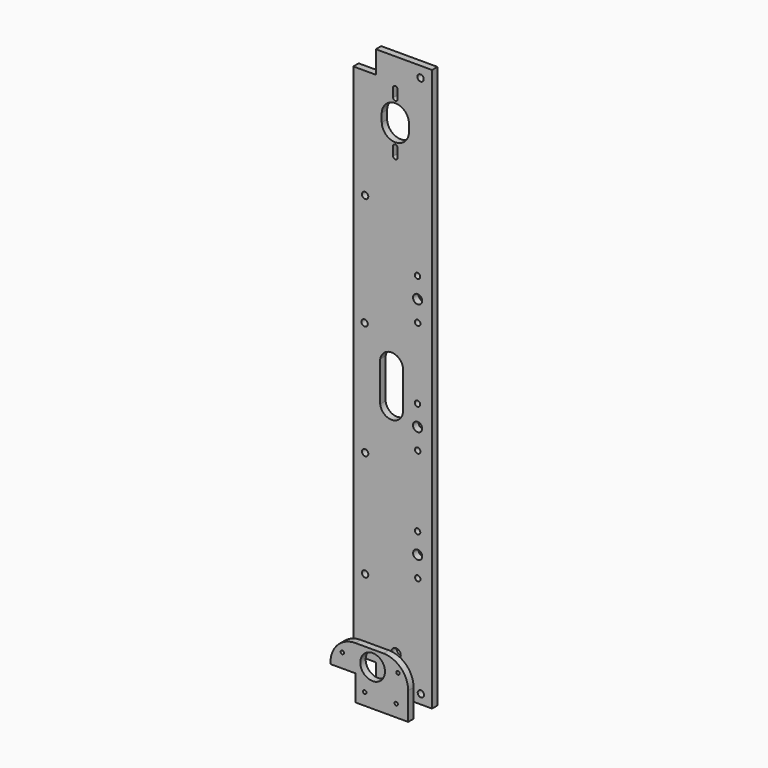
from build123d import *

# Parameters (mm, degrees)
F0_R     = 2.8321056642
F0_R_2   = 2.8346456693
F0_R_3   = 4.2506985014
F0_R_4   = 2.4282448565
F0_R_5   = 4.0601981204
F0_R_6   = 2.4234188468
F0_R_7   = 2.8384556769
F0_R_8   = 2.8333756668
F1_DEPTH = 6
F3_R     = 1.5196800403
F3_R_2   = 1.5209496142
F3_R_3   = 11
F4_DEPTH = 6


# Not quite as in the source:
# - ends of sketch curves that miss each other by under 0.0002 mm in the source are joined


with BuildPart() as f1:
    # F0 (on Front) → F1 (new body)
    with BuildSketch(Plane.XZ):
        Polygon((-15.0012700025, 250), (-15.0012700025, 230), (-34.9987299975, 230), (-34.9987299975, -230), (-15.0012700025, -230), (-15.0012700025, -250), (34.9987299975, -250), (34.9987299975, 250), align=None)
        with Locations((-24.5161290323, -163.967487935)):
            Circle(F0_R, mode=Mode.SUBTRACT)
        with Locations((-24.5161290323, -68.9585979172)):
            Circle(F0_R_2, mode=Mode.SUBTRACT)
        with BuildLine():
            ThreePointArc((-11.0922101342, 8.6664987085), (-0.9906019812, 17.1704343409), (9.1110061718, 8.6664987085))
            Line((9.1110061718, 8.6664987085), (9.110998222, -26.6289052578))
            ThreePointArc((9.110998222, -26.6289052578), (-0.9906019812, -35.5824231648), (-11.0922037581, -26.6289054481))
            Line((-11.0922037581, -26.6289054481), (-11.0922101342, 8.6664987085))
        make_face(mode=Mode.SUBTRACT)
        with Locations((2.9337058674, -217.3037846076)):
            Circle(F0_R_3, mode=Mode.SUBTRACT)
        with Locations((25.0952501905, -241.6408432817)):
            Circle(F0_R_2, mode=Mode.SUBTRACT)
        with Locations((22.3344424689, -152.1221742443)):
            Circle(F0_R_4, mode=Mode.SUBTRACT)
        with Locations((22.2428244856, -133.6652273305)):
            Circle(F0_R_5, mode=Mode.SUBTRACT)
        with Locations((22.1522987046, -115.4320548641)):
            Circle(F0_R_6, mode=Mode.SUBTRACT)
        with Locations((22.2455422911, -52.1094742189)):
            Circle(F0_R_4, mode=Mode.SUBTRACT)
        with Locations((22.1539243078, -33.6525273051)):
            Circle(F0_R_5, mode=Mode.SUBTRACT)
        with Locations((22.0633985268, -15.4193548387)):
            Circle(F0_R_6, mode=Mode.SUBTRACT)
        with Locations((-24.953009906, 32.4752349505)):
            Circle(F0_R_7, mode=Mode.SUBTRACT)
        with Locations((-24.5161290323, 132.3888747777)):
            Circle(F0_R_8, mode=Mode.SUBTRACT)
        with Locations((22.2455422911, 47.904495809)):
            Circle(F0_R_4, mode=Mode.SUBTRACT)
        with Locations((22.1539243078, 66.3614427229)):
            Circle(F0_R_5, mode=Mode.SUBTRACT)
        with Locations((22.0633985268, 84.5946151892)):
            Circle(F0_R_6, mode=Mode.SUBTRACT)
        with BuildLine():
            ThreePointArc((0.322589783, 179.2583173603), (2.3685547371, 181.0616967234), (4.4145196912, 179.2583173603))
            Line((4.4145196912, 179.2583173603), (4.4145288291, 171.2014224028))
            ThreePointArc((4.4145288291, 171.2014224028), (2.3685547371, 169.395478791), (0.3225807849, 171.2014224203))
            Line((0.3225807849, 171.2014224203), (0.322589783, 179.2583173603))
        make_face(mode=Mode.SUBTRACT)
        with BuildLine():
            ThreePointArc((-9.7358355642, 201.8008634341), (2.3672847346, 213.3959613919), (14.4704050333, 201.8008634341))
            Line((14.4704050333, 201.8008634341), (14.4704089408, 194.3281686563))
            ThreePointArc((14.4704089408, 194.3281686563), (2.3672847346, 182.730480061), (-9.735849035, 194.3281682483))
            Line((-9.735849035, 194.3281682483), (-9.7358355642, 201.8008634341))
        make_face(mode=Mode.SUBTRACT)
        with BuildLine():
            ThreePointArc((0.322589783, 225.0952490342), (2.3685547371, 226.8986283973), (4.4145196912, 225.0952490342))
            Line((4.4145196912, 225.0952490342), (4.4145288291, 217.0383540767))
            ThreePointArc((4.4145288291, 217.0383540767), (2.3685547371, 215.2324104648), (0.3225807849, 217.0383540942))
            Line((0.3225807849, 217.0383540942), (0.322589783, 225.0952490342))
        make_face(mode=Mode.SUBTRACT)
        with Locations((24.7548895098, 240.3987807976)):
            Circle(F0_R_2, mode=Mode.SUBTRACT)
    extrude(amount=F1_DEPTH)


with BuildPart() as f4:
    # F3 (on offset) → F4 (new body)
    with BuildSketch(Plane.XZ.offset(26)):
        with BuildLine():
            Line((-34.429923848, -225.4829136519), (-34.429923848, -227.1858596432))
            Line((-34.429923848, -227.1858596432), (-12.0509845344, -227.1858596432))
            Line((-12.0509845344, -227.1858596432), (-12.0509845344, -249.9848689689))
            Line((-12.0509845344, -249.9848689689), (34.579038782, -249.9848689689))
            Line((34.579038782, -249.9848689689), (34.579038782, -225.4829136519))
            ThreePointArc((34.579038782, -225.4829136519), (28.1353879681, -209.9265644658), (12.579038782, -203.4829136519))
            Line((12.579038782, -203.4829136519), (-12.429923848, -203.4829136519))
            ThreePointArc((-12.429923848, -203.4829136519), (-27.9862730341, -209.9265644658), (-34.429923848, -225.4829136519))
        make_face()
        with Locations((-4.0056942962, -239.2163425684)):
            Circle(F3_R, mode=Mode.SUBTRACT)
        with Locations((23.9438176482, -239.2163425684)):
            Circle(F3_R, mode=Mode.SUBTRACT)
        with Locations((-24.0575045256, -214.5586769528)):
            Circle(F3_R_2, mode=Mode.SUBTRACT)
        with Locations((2.9655364342, -217.3086702824)):
            Circle(F3_R_3, mode=Mode.SUBTRACT)
        with Locations((25.5461439863, -214.5586769528)):
            Circle(F3_R, mode=Mode.SUBTRACT)
    extrude(amount=F4_DEPTH)


solid = Compound([f1.part, f4.part])
